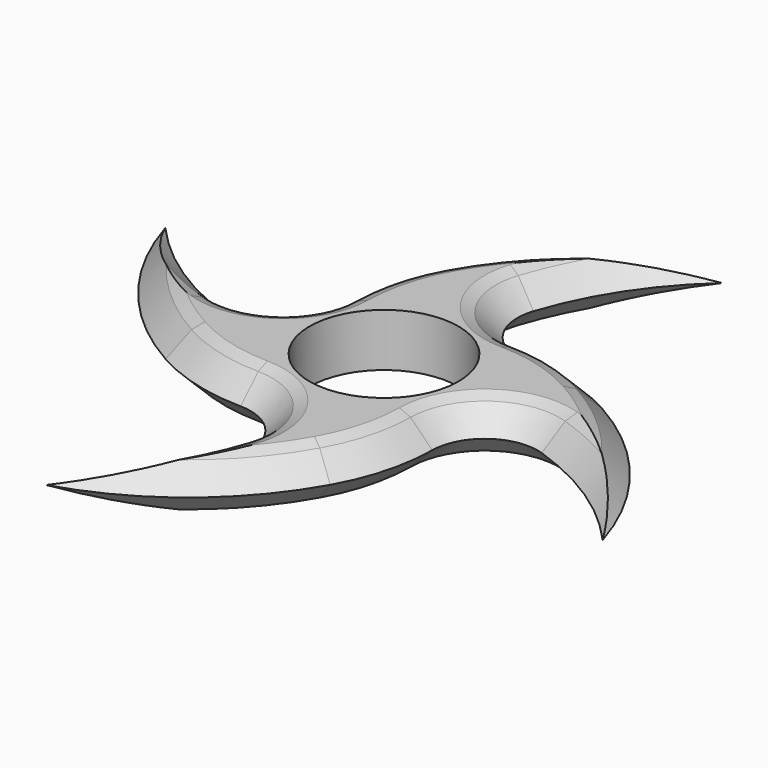
from build123d import *

# Parameters (mm, degrees)
F1_DEPTH = 203.2
F2_R     = 762
F3_R     = 203.2
F4_SIZE  = 101.5999
F5_SIZE  = 25.4


# Not quite as in the source:
# - a fillet or chamfer is up to 0.001 mm smaller than in the source, because OpenCascade refuses the exact size


with BuildPart() as f1:
    # F0 (on Top) → F1 (new body)
    with BuildSketch(Plane.XY):
        with BuildLine():
            Line((381, -381), (0, -381))
            ThreePointArc((0, -381), (-116.8520700538, -798.8239649731), (-381, -1143))
            ThreePointArc((-381, -1143), (95.4373187158, -857.4373187158), (381, -381))
        make_face()
        with BuildLine():
            Line((-381, -381), (-381, 0))
            ThreePointArc((-381, 0), (-798.8239649731, 116.8520700538), (-1143, 381))
            ThreePointArc((-1143, 381), (-857.4373187158, -95.4373187158), (-381, -381))
        make_face()
        with BuildLine():
            Line((-381, 381), (0, 381))
            ThreePointArc((0, 381), (116.8520700538, 798.8239649731), (381, 1143))
            ThreePointArc((381, 1143), (-95.4373187158, 857.4373187158), (-381, 381))
        make_face()
        with BuildLine():
            Line((381, 381), (381, 0))
            ThreePointArc((381, 0), (798.8239649731, -116.8520700538), (1143, -381))
            ThreePointArc((1143, -381), (857.4373187158, 95.4373187158), (381, 381))
        make_face()
        with BuildLine():
            Line((381, 381), (0, 381))
            ThreePointArc((0, 381), (269.4076836321, 269.4076836321), (381, 0))
            Line((381, 0), (381, 381))
        make_face()
        with BuildLine():
            ThreePointArc((-381, 0), (-269.4076836321, 269.4076836321), (0, 381))
            Line((0, 381), (-381, 381))
            Line((-381, 381), (-381, 0))
        make_face()
        with BuildLine():
            ThreePointArc((381, 0), (269.4076836321, 269.4076836321), (0, 381))
            ThreePointArc((0, 381), (-269.4076836321, 269.4076836321), (-381, 0))
            ThreePointArc((-381, 0), (-269.4076836321, -269.4076836321), (0, -381))
            ThreePointArc((0, -381), (269.4076836321, -269.4076836321), (381, 0))
        make_face()
        with BuildLine():
            ThreePointArc((0, 292.1), (206.5458907846, 206.5458907846), (292.1, 0))
            ThreePointArc((292.1, 0), (-206.5458907846, -206.5458907846), (0, 292.1))
        make_face(mode=Mode.SUBTRACT)
        with BuildLine():
            ThreePointArc((0, -381), (-269.4076836321, -269.4076836321), (-381, 0))
            Line((-381, 0), (-381, -381))
            Line((-381, -381), (0, -381))
        make_face()
        with BuildLine():
            Line((381, -381), (381, 0))
            ThreePointArc((381, 0), (269.4076836321, -269.4076836321), (0, -381))
            Line((0, -381), (381, -381))
        make_face()
        with BuildLine():
            ThreePointArc((0, 292.1), (-206.5458907846, -206.5458907846), (292.1, 0))
            ThreePointArc((292.1, 0), (206.5458907846, 206.5458907846), (0, 292.1))
        make_face()
        with BuildLine():
            ThreePointArc((285.75, 0), (-202.0557627241, -202.0557627241), (0, 285.75))
            ThreePointArc((0, 285.75), (202.0557627241, 202.0557627241), (285.75, 0))
        make_face(mode=Mode.SUBTRACT)
    extrude(amount=F1_DEPTH)

    # F2
    f2_edges = [f1.edges().sort_by_distance(p)[0] for p in [
        (381, 381, 101.6),
        (-381, 381, 101.6),
        (-381, -381, 101.6),
        (381, -381, 101.6),
    ]]
    fillet(f2_edges, radius=F2_R)

    # F3
    f3_edges = [f1.edges().sort_by_distance(p)[0] for p in [
        (-381, 0, 101.6),
        (0, -381, 101.6),
        (381, 0, 101.6),
        (0, 381, 101.6),
    ]]
    fillet(f3_edges, radius=F3_R)

    # F4 (size 101.6 in the source; OpenCascade refuses exactly that, so slightly less here)
    f4_edges = [f1.edges().sort_by_distance(p)[0] for p in [
        (185.144546, 917.151375, 203.2),
        (185.144546, 917.151375, 0),
        (-185.144546, -917.151375, 0),
        (-185.144546, -917.151375, 203.2),
        (-917.151375, 185.144546, 203.2),
        (-917.151375, 185.144546, 0),
        (466.189412, -81.909659, 203.2),
        (466.189412, -81.909659, 0),
    ]]
    chamfer(f4_edges, length=F4_SIZE)

    # F5
    f5_edges = [f1.edges().sort_by_distance(p)[0] for p in [
        (407.214739, 0.822007, 203.2),
        (407.933051, 256.763283, 203.2),
        (0.822007, -407.214739, 203.2),
        (-407.214739, -0.822007, 203.2),
        (-407.214739, -0.822007, 0),
        (-407.933051, -256.763283, 0),
        (256.763283, -407.933051, 0),
        (-0.822007, 407.214739, 0),
    ]]
    chamfer(f5_edges, length=F5_SIZE)


solid = f1.part
